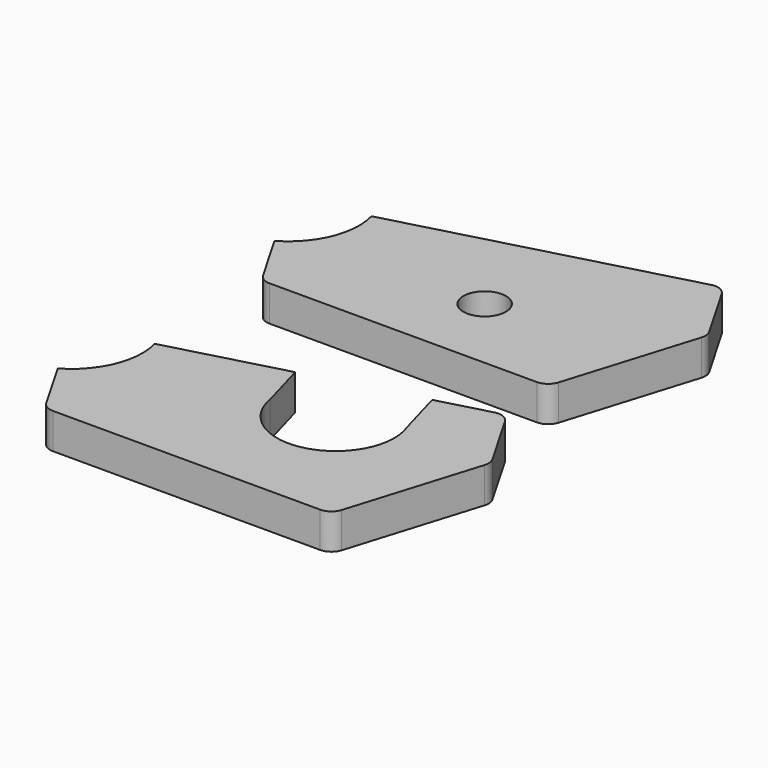
from build123d import *

# Parameters (mm, degrees)
F0_R     = 3
F1_DEPTH = 5
F2_DEPTH = 5


# Not quite as in the source:
# - ends of sketch curves that miss each other by under 0.0002 mm in the source are joined


with BuildPart() as f1:
    # F0 (on Top) → F1 (new body)
    with BuildSketch(Plane.XY):
        with BuildLine():
            Line((-9.888975, 25.438376), (-14.465956, 33.365941))
            ThreePointArc((-14.465956, 33.365941), (-15.4331378873, 34.2139061621), (-16.71668586, 34.2975134786))
            Line((-16.71668586, 34.2975134786), (-56.088806, 23.725041))
            ThreePointArc((-56.088806, 23.725041), (-56.5082159612, 17.3088367317), (-60.7474589836, 12.4743359716))
            Line((-60.7474589836, 12.4743359716), (-56.574809, 5.247095))
            ThreePointArc((-56.574809, 5.247095), (-55.8427580417, 4.5150442165), (-54.842758, 4.247095))
            Line((-54.842758, 4.247095), (-17.208055, 4.247095))
            ThreePointArc((-17.208055, 4.247095), (-16.019435709, 4.6386223763), (-15.2961934105, 5.6599108189))
            Line((-15.2961934105, 5.6599108189), (-9.709164, 23.851193))
            ThreePointArc((-9.709164, 23.851193), (-9.633738266, 24.6635147626), (-9.888975, 25.438376))
        make_face()
        with Locations((-33.32098, 15.198094)):
            Circle(F0_R, mode=Mode.SUBTRACT)
    extrude(amount=F1_DEPTH)


with BuildPart() as f2:
    # F0 (on Top) → F2 (new body)
    with BuildSketch(Plane.XY):
        with BuildLine():
            Line((-16.353472, -4.315521), (-23.554763, -6.249261))
            Line((-23.554763, -6.249261), (-21.665791, -12.990118))
            ThreePointArc((-21.665791, -12.990118), (-27.2335281118, -23.941313877), (-37.5470821174, -17.2660610188))
            Line((-37.5470821174, -17.2660610188), (-39.44013, -10.514909))
            Line((-39.44013, -10.514909), (-55.725593, -14.887994))
            ThreePointArc((-55.725593, -14.887994), (-56.1450019117, -21.3041981487), (-60.3842449836, -26.1386990284))
            Line((-60.3842449836, -26.1386990284), (-56.211595, -33.36594))
            ThreePointArc((-56.211595, -33.36594), (-55.4795440417, -34.0979907835), (-54.479544, -34.36594))
            Line((-54.479544, -34.36594), (-16.844842, -34.36594))
            ThreePointArc((-16.844842, -34.36594), (-15.6562225909, -33.9744125364), (-14.9329803243, -32.9531239004))
            Line((-14.9329803243, -32.9531239004), (-9.34595, -14.761842))
            ThreePointArc((-9.34595, -14.761842), (-9.2705242122, -13.9495197123), (-9.5257611443, -13.1746580833))
            Line((-9.5257611443, -13.1746580833), (-14.102742, -5.247094))
            ThreePointArc((-14.102742, -5.247094), (-15.0699238873, -4.3991288379), (-16.353472, -4.315521))
        make_face()
    extrude(amount=F2_DEPTH)


solid = Compound([f1.part, f2.part])
